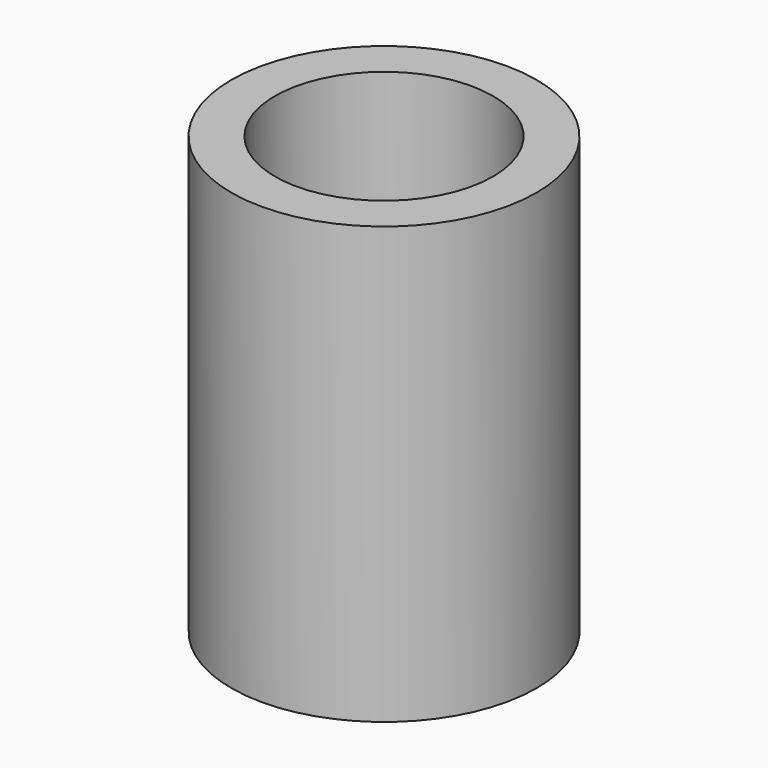
from build123d import *

# Parameters (mm, degrees)
F0_R     = 8.89
F1_DEPTH = 25.4
F2_R     = 6.35
F3_DEPTH = 34.8742


# Not quite as in the source:
# - the program builds the solid bodies; features that only make, move or delete a surface that nothing else refers to are left out


with BuildPart() as f1:
    # F0 (on Top) → F1 (new body)
    with BuildSketch(Plane.XY):
        Circle(F0_R)
    extrude(amount=F1_DEPTH)

    # F2 (on face) → F3 (cut)
    with BuildSketch(Plane.XY.offset(25.4)):
        Circle(F2_R)
    extrude(amount=-F3_DEPTH, mode=Mode.SUBTRACT)


solid = f1.part
